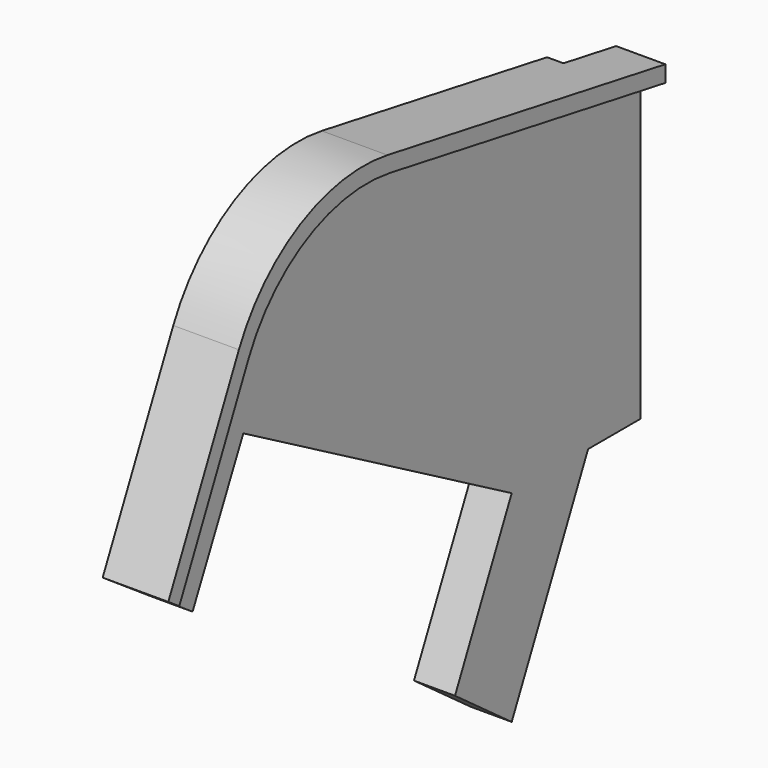
from build123d import *

# Parameters (mm, degrees)
F1_DEPTH = 5
F3_DEPTH = 3
F4_R     = 20
F5_R     = 21
F7_DEPTH = 2


with BuildPart() as f1:
    # F0 (on Right) → F1 (new body)
    with BuildSketch(Plane.YZ):
        Polygon((-2.6435090923, -26.501225133), (5.3746857459, -26.501225133), (5.3746857459, -16.4436940104), (-55.1649013234, -3.4599144195), (-14.2791476101, -26.501225133), (-22.9189545176, -44.7233500122), (-14.2791476101, -51.0418266058), align=None)
        Polygon((-55.1649013234, -3.4599144195), (5.3746857459, -16.4436940104), (5.3746857459, 12.498774867), (-52.7289716819, 22.7440173494), (-70.3398138285, -14.3988225609), (-62.8945189948, -19.4552624983), align=None)
    extrude(amount=F1_DEPTH)

    # F2 (on face) → F3 (join)
    with BuildSketch(Plane.YZ.offset(5)):
        Polygon((5.3746857459, 12.498774867), (-52.7289716819, 22.7440173494), (-70.3398138285, -14.3988225609), (-68.6655286126, -15.5359061582), (-51.5614379211, 20.5381496464), (5.3746857459, 10.498774867), align=None)
    extrude(amount=F3_DEPTH)

    # F4
    f4_edges = [f1.edges().sort_by_distance(p)[0] for p in [
        (6.5, -51.561438, 20.53815),
    ]]
    fillet(f4_edges, radius=F4_R)

    # F5
    f5_edges = [f1.edges().sort_by_distance(p)[0] for p in [
        (4, -52.728972, 22.744017),
    ]]
    fillet(f5_edges, radius=F5_R)

    # F6 (on face) → F7 (cut)
    with BuildSketch(Plane(origin=(0, 0, 0), x_dir=(0, -1, 0), z_dir=(-1, 0, 0))):
        Polygon((2.6435090923, 13.9125989535), (-5.3746857459, 12.498774867), (-5.3746857459, -26.501225133), (2.6435090923, -26.501225133), align=None)
    extrude(amount=-F7_DEPTH, mode=Mode.SUBTRACT)


solid = f1.part
